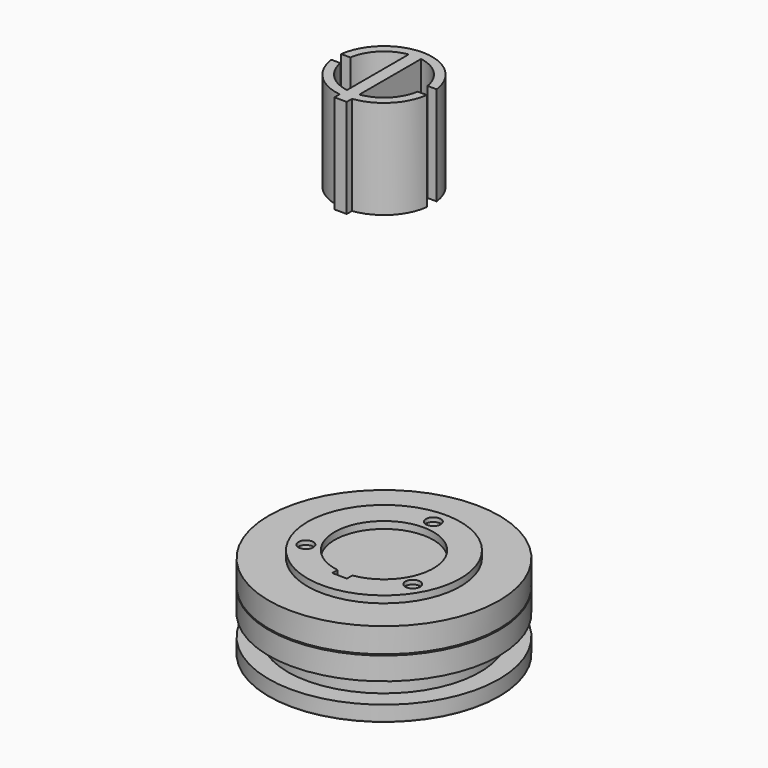
from build123d import *

# Parameters (mm, degrees)
F7_R      = 14
F8_DEPTH  = 0.55
F10_DEPTH = 1
F11_W     = 1.5
F11_H     = 7.8581168228
F12_DEPTH = 1.55
F19_DEPTH = 12
F20_R     = 1
F24_DEPTH = 2.4
F26_DEPTH = 2.1
F28_DEPTH = 11
F30_DEPTH = 12
F31_R     = 0.9
F32_DEPTH = 0.5


with BuildPart() as f8:
    # F7 (on Top) → F8 (new body)
    with BuildSketch(Plane.XY):
        Circle(F7_R)
    extrude(amount=F8_DEPTH)

    # F9 (on face) → F10 (join)
    with BuildSketch(Plane.XY.offset(0.55)):
        with BuildLine():
            Line((0.6, -6.6), (0.6, -5.9699246226))
            ThreePointArc((0.6, -5.9699246226), (0, 6), (-0.6, -5.9699246226))
            Line((-0.6, -5.9699246226), (-0.6, -6.6))
            Line((-0.6, -6.6), (0.6, -6.6))
        make_face()
    extrude(amount=F10_DEPTH)

    # F11 (on face) → F12 (cut, through all)
    with BuildSketch(Plane.XY.offset(1.55)):
        Rectangle(F11_W, F11_H)
    extrude(amount=-F12_DEPTH, mode=Mode.SUBTRACT)


with BuildPart() as f14:
    # F13 (on Front) → F14 (revolve)
    with BuildSketch(Plane.XZ):
        Polygon((-9.675, 7.1), (-14, 7.1), (-14, 4.35), (-11.675, 4.35), (-11.675, 1.85), (-14, 1.85), (-14, 1.1), (-14, 0.1), (-9.675, 0.1), (-6.15, 0.1), (-6.15, 1.1), (-9.675, 1.1), align=None)
    revolve(axis=Axis((0, 0, 0.110375745), (0, 0, -1)))

    # F23 (on face) → F24 (cut)
    with BuildSketch(Plane.XY.offset(7.1)):
        with BuildLine():
            ThreePointArc((-2.4, -10.7606052339), (0, -11.025), (2.4, -10.7606052339))
            Line((2.4, -10.7606052339), (2.4, -9.3725996927))
            ThreePointArc((2.4, -9.3725996927), (0, -9.675), (-2.4, -9.3725996927))
            Line((-2.4, -9.3725996927), (-2.4, -10.7606052339))
        make_face()
    extrude(amount=-F24_DEPTH, mode=Mode.SUBTRACT)


with BuildPart() as f16:
    # F15 (on Front) → F16 (revolve)
    with BuildSketch(Plane.XZ):
        Polygon((0, 10.25), (-14, 10.25), (-14, 7.25), (-10, 7.25), (-10, 9.25), (0, 9.25), align=None)
    revolve(axis=Axis((0, 0, 0.110375745), (0, 0, -1)))


with BuildPart() as f19:
    # F18 (on offset) → F19 (new body)
    with BuildSketch(Plane.XY.offset(50)):
        with BuildLine():
            Line((-4.6904157598, -0.75), (-5.8017238817, -0.75))
            ThreePointArc((-5.8017238817, -0.75), (0, -5.85), (5.8017238817, -0.75))
            Line((5.8017238817, -0.75), (4.6904157598, -0.75))
            ThreePointArc((4.6904157598, -0.75), (3.3587572106, -3.3587572106), (0.75, -4.6904157598))
            Line((0.75, -4.6904157598), (0.75, 4.6904157598))
            ThreePointArc((0.75, 4.6904157598), (3.3587572106, 3.3587572106), (4.6904157598, 0.75))
            Line((4.6904157598, 0.75), (5.8017238817, 0.75))
            ThreePointArc((5.8017238817, 0.75), (0, 5.85), (-5.8017238817, 0.75))
            Line((-5.8017238817, 0.75), (-4.6904157598, 0.75))
            ThreePointArc((-4.6904157598, 0.75), (-3.3587572106, 3.3587572106), (-0.75, 4.6904157598))
            Line((-0.75, 4.6904157598), (-0.75, -4.6904157598))
            ThreePointArc((-0.75, -4.6904157598), (-3.3587572106, -3.3587572106), (-4.6904157598, -0.75))
        make_face()
    extrude(amount=F19_DEPTH)

    # F29 (on face) → F30 (join)
    with BuildSketch(Plane.XY.offset(62)):
        with BuildLine():
            Line((-0.75, -6.6), (0.75, -6.6))
            Line((0.75, -6.6), (0.75, -5.8017238817))
            ThreePointArc((0.75, -5.8017238817), (0, -5.85), (-0.75, -5.8017238817))
            Line((-0.75, -5.8017238817), (-0.75, -6.6))
        make_face()
    extrude(amount=-F30_DEPTH)


with BuildPart() as f21:
    # F20 (on Front) → F21 (revolve)
    with BuildSketch(Plane.XZ):
        with BuildLine():
            Line((-6, 11.1), (-9.3035714286, 11.1))
            Line((-9.3035714286, 11.1), (-9.3035714286, 10.1))
            Line((-9.3035714286, 10.1), (-8.375, 10.1))
            ThreePointArc((-8.375, 10.1), (-8.0214466094, 9.9535533906), (-7.875, 9.6))
            Line((-7.875, 9.6), (-7.875, 8.85))
            Line((-7.875, 8.85), (-7.875, 8.1))
            ThreePointArc((-7.875, 8.1), (-8.0214466094, 7.7464466094), (-8.375, 7.6))
            Line((-8.375, 7.6), (-9.3035714286, 7.6))
            Line((-9.3035714286, 7.6), (-9.3035714286, 4.6))
            Line((-9.3035714286, 4.6), (-8.375, 4.6))
            ThreePointArc((-8.375, 4.6), (-8.0214466094, 4.4535533906), (-7.875, 4.1))
            Line((-7.875, 4.1), (-7.875, 3.35))
            Line((-7.875, 3.35), (-7.875, 2.6))
            ThreePointArc((-7.875, 2.6), (-8.0214466094, 2.2464466094), (-8.375, 2.1))
            Line((-8.375, 2.1), (-9.3035714286, 2.1))
            Line((-9.3035714286, 2.1), (-9.3035714286, 1.1))
            Line((-9.3035714286, 1.1), (-6, 1.1))
            Line((-6, 1.1), (-6, 11.1))
        make_face()
    revolve(axis=Axis((0, 0, 4.9723982811), (0, 0, -1)))

    # F25 (on face) → F26 (join)
    with BuildSketch(Plane.XY.offset(7.1)):
        with BuildLine():
            Line((-2.25, -5.5621488653), (-2.25, -10.6396957193))
            ThreePointArc((-2.25, -10.6396957193), (0, -10.875), (2.25, -10.6396957193))
            Line((2.25, -10.6396957193), (2.25, -5.5621488653))
            ThreePointArc((2.25, -5.5621488653), (0, -6), (-2.25, -5.5621488653))
        make_face()
    extrude(amount=-F26_DEPTH)


with BuildPart() as f22:
    # F20 (on Front) → F22 (revolve)
    with BuildSketch(Plane.XZ):
        with Locations((-8.875, 8.85)):
            Circle(F20_R)
    revolve(axis=Axis((0, 0, 4.9723982811), (0, 0, -1)))


with BuildPart() as f22b:
    # F20 (on Front) → F22, piece 2 (revolve)
    with BuildSketch(Plane.XZ):
        with Locations((-8.875, 3.35)):
            Circle(F20_R)
    revolve(axis=Axis((0, 0, 4.9723982811), (0, 0, -1)))


with BuildPart() as f28_tool:
    # F27 (on face) → F28 (new body, through all)
    with BuildSketch(Plane.XY.offset(11.1)):
        with BuildLine():
            Line((-0.9, -6.7316994618), (0.9, -6.7686159747))
            Line((0.9, -6.7686159747), (0.9, -5.93211598))
            ThreePointArc((0.9, -5.93211598), (0, -6), (-0.9, -5.93211598))
            Line((-0.9, -5.93211598), (-0.9, -6.7316994618))
        make_face()
    extrude(amount=-F28_DEPTH)


with BuildPart() as f14_1:
    add(f14.part)

    # F28: cut by f28_tool
    add(f28_tool.part, mode=Mode.SUBTRACT)


with BuildPart() as f21_1:
    add(f21.part)

    # F28: cut by f28_tool
    add(f28_tool.part, mode=Mode.SUBTRACT)

    # F31 (on face) → F32 (cut)
    with BuildSketch(Plane.XY.offset(11.1)):
        with Locations((0, 7.5)):
            Circle(F31_R)
        with Locations((6.4951905374, -3.7499999845)):
            Circle(F31_R)
        with Locations((-6.4951905104, -3.7500000311)):
            Circle(F31_R)
    extrude(amount=-F32_DEPTH, mode=Mode.SUBTRACT)


solid = Compound([f8.part, f16.part, f19.part, f22.part, f22b.part, f14_1.part, f21_1.part])
